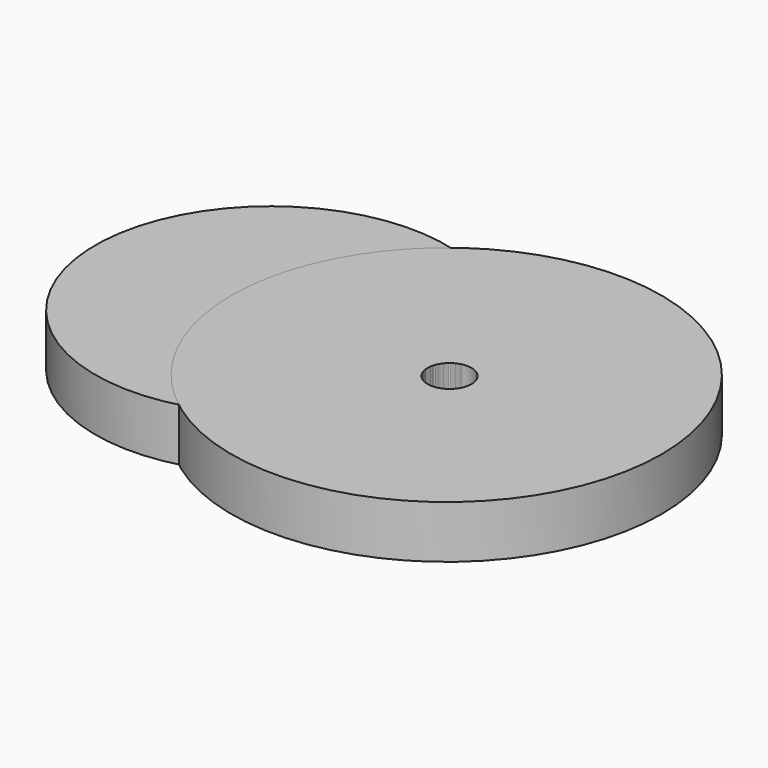
from build123d import *

# Parameters (mm, degrees)
F0_R     = 20
F1_DEPTH = 6
F4_R     = 24.5
F5_DEPTH = 6
F8_D     = 5
F8_2_D   = 5


# Not quite as in the source:
# - a feature of the source that left no trace in its solid (it failed there, or was rolled back) is left out
# - the program builds the solid bodies; features that only make, move or delete a surface that nothing else refers to are left out


with BuildPart() as f1:
    # F0 (on Top) → F1 (new body)
    with BuildSketch(Plane.XY):
        Circle(F0_R)
    extrude(amount=F1_DEPTH)

    # F8 (through all)
    with Locations(Plane(origin=(0, 0, 0), x_dir=(1, 0, 0), z_dir=(0, 0, -1))):
        with Locations((20.3447919339, 0)):
            Hole(F8_D / 2)


with BuildPart() as f5:
    # F4 (on Top) → F5 (new body)
    with BuildSketch(Plane.XY):
        with Locations((20, 0)):
            Circle(F4_R)
    extrude(amount=F5_DEPTH)

    # F8#2 (through all)
    with Locations(Plane(origin=(0, 0, 0), x_dir=(1, 0, 0), z_dir=(0, 0, -1))):
        with Locations((20.3447919339, 0)):
            Hole(F8_2_D / 2)


solid = Compound([f1.part, f5.part])
